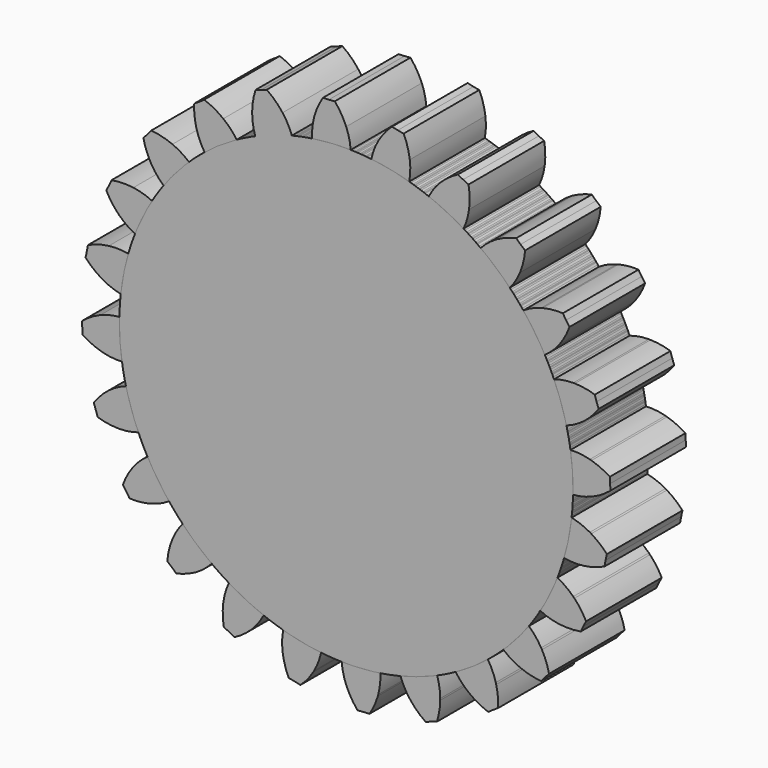
from build123d import *

# Parameters (mm, degrees)
F1_DEPTH = 25
F2_COUNT = 24
F2_ANGLE = 345


with BuildPart() as f1:
    # F0 (on Front) → F1 (new body)
    with BuildSketch(Plane.XZ):
        with BuildLine():
            ThreePointArc((-9.0111976673, 59.3194598475), (-39.1109200861, -45.5009442761), (60, 0))
            ThreePointArc((60, 0), (42.845546701, 42.0030847426), (1.1913624036, 59.9881709641))
            ThreePointArc((1.1913624036, 59.9881709641), (-1.3676565953, 59.9844106034), (-3.9241877538, 59.8715353943))
            ThreePointArc((-3.9241877538, 59.8715353943), (-6.4735806051, 59.6497506629), (-9.0111976673, 59.3194598475))
        make_face()
        with BuildLine():
            ThreePointArc((-8.4842024943, 64.4439159893), (-8.9485442404, 61.9023425791), (-9.0111976673, 59.3194598475))
            ThreePointArc((-9.0111976673, 59.3194598475), (-6.4735806051, 59.6497506629), (-3.9241877538, 59.8715353943))
            Line((-3.9241877538, 59.8715353943), (-4.2559103924, 64.9326448372))
            Line((-4.2559103924, 64.9326448372), (-8.3665646405, 64.8675885366))
            ThreePointArc((-8.3665646405, 64.8675885366), (-8.4266447953, 64.6561024583), (-8.4842024943, 64.4439159893))
        make_face()
        with BuildLine():
            Line((-8.3665646405, 64.8675885366), (-4.2559103924, 64.9326448372))
            Line((-4.2559103924, 64.9326448372), (-4.5749731638, 69.8006020322))
            ThreePointArc((-4.5749731638, 69.8006020322), (-5.361514281, 69.7570438044), (-6.1487762364, 69.7294238524))
            ThreePointArc((-6.1487762364, 69.7294238524), (-7.4344903349, 67.3791648533), (-8.3665646405, 64.8675885366))
        make_face()
        with BuildLine():
            Line((-4.2559103924, 64.9326448372), (0, 65))
            ThreePointArc((0, 65), (-1.3083979526, 67.5860266971), (-3.0053435778, 69.935455314))
            ThreePointArc((-3.0053435778, 69.935455314), (-3.7894755253, 69.8600806681), (-4.5749731638, 69.8006020322))
            Line((-4.5749731638, 69.8006020322), (-4.2559103924, 64.9326448372))
        make_face()
        with BuildLine():
            ThreePointArc((-3.9241877538, 59.8715353943), (-1.3676565953, 59.9844106034), (1.1913624036, 59.9881709641))
            ThreePointArc((1.1913624036, 59.9881709641), (0.7921111376, 62.5407788626), (0, 65))
            Line((0, 65), (-4.2559103924, 64.9326448372))
            Line((-4.2559103924, 64.9326448372), (-3.9241877538, 59.8715353943))
        make_face()
    extrude(amount=F1_DEPTH)


with BuildPart() as f2_1:
    # F2: instance of F1
    add(f1.part.rotate(Axis((0, -25, 0), (0, 1, 0)), 1 * F2_ANGLE / (F2_COUNT - 1)))


with BuildPart() as f2_2:
    # F2: instance of F1
    add(f1.part.rotate(Axis((0, -25, 0), (0, 1, 0)), 2 * F2_ANGLE / (F2_COUNT - 1)))


with BuildPart() as f2_3:
    # F2: instance of F1
    add(f1.part.rotate(Axis((0, -25, 0), (0, 1, 0)), 3 * F2_ANGLE / (F2_COUNT - 1)))


with BuildPart() as f2_4:
    # F2: instance of F1
    add(f1.part.rotate(Axis((0, -25, 0), (0, 1, 0)), 4 * F2_ANGLE / (F2_COUNT - 1)))


with BuildPart() as f2_5:
    # F2: instance of F1
    add(f1.part.rotate(Axis((0, -25, 0), (0, 1, 0)), 5 * F2_ANGLE / (F2_COUNT - 1)))


with BuildPart() as f2_6:
    # F2: instance of F1
    add(f1.part.rotate(Axis((0, -25, 0), (0, 1, 0)), 6 * F2_ANGLE / (F2_COUNT - 1)))


with BuildPart() as f2_7:
    # F2: instance of F1
    add(f1.part.rotate(Axis((0, -25, 0), (0, 1, 0)), 7 * F2_ANGLE / (F2_COUNT - 1)))


with BuildPart() as f2_8:
    # F2: instance of F1
    add(f1.part.rotate(Axis((0, -25, 0), (0, 1, 0)), 8 * F2_ANGLE / (F2_COUNT - 1)))


with BuildPart() as f2_9:
    # F2: instance of F1
    add(f1.part.rotate(Axis((0, -25, 0), (0, 1, 0)), 9 * F2_ANGLE / (F2_COUNT - 1)))


with BuildPart() as f2_10:
    # F2: instance of F1
    add(f1.part.rotate(Axis((0, -25, 0), (0, 1, 0)), 10 * F2_ANGLE / (F2_COUNT - 1)))


with BuildPart() as f2_11:
    # F2: instance of F1
    add(f1.part.rotate(Axis((0, -25, 0), (0, 1, 0)), 11 * F2_ANGLE / (F2_COUNT - 1)))


with BuildPart() as f2_12:
    # F2: instance of F1
    add(f1.part.rotate(Axis((0, -25, 0), (0, 1, 0)), 12 * F2_ANGLE / (F2_COUNT - 1)))


with BuildPart() as f2_13:
    # F2: instance of F1
    add(f1.part.rotate(Axis((0, -25, 0), (0, 1, 0)), 13 * F2_ANGLE / (F2_COUNT - 1)))


with BuildPart() as f2_14:
    # F2: instance of F1
    add(f1.part.rotate(Axis((0, -25, 0), (0, 1, 0)), 14 * F2_ANGLE / (F2_COUNT - 1)))


with BuildPart() as f2_15:
    # F2: instance of F1
    add(f1.part.rotate(Axis((0, -25, 0), (0, 1, 0)), 15 * F2_ANGLE / (F2_COUNT - 1)))


with BuildPart() as f2_16:
    # F2: instance of F1
    add(f1.part.rotate(Axis((0, -25, 0), (0, 1, 0)), 16 * F2_ANGLE / (F2_COUNT - 1)))


with BuildPart() as f2_17:
    # F2: instance of F1
    add(f1.part.rotate(Axis((0, -25, 0), (0, 1, 0)), 17 * F2_ANGLE / (F2_COUNT - 1)))


with BuildPart() as f2_18:
    # F2: instance of F1
    add(f1.part.rotate(Axis((0, -25, 0), (0, 1, 0)), 18 * F2_ANGLE / (F2_COUNT - 1)))


with BuildPart() as f2_19:
    # F2: instance of F1
    add(f1.part.rotate(Axis((0, -25, 0), (0, 1, 0)), 19 * F2_ANGLE / (F2_COUNT - 1)))


with BuildPart() as f2_20:
    # F2: instance of F1
    add(f1.part.rotate(Axis((0, -25, 0), (0, 1, 0)), 20 * F2_ANGLE / (F2_COUNT - 1)))


with BuildPart() as f2_21:
    # F2: instance of F1
    add(f1.part.rotate(Axis((0, -25, 0), (0, 1, 0)), 21 * F2_ANGLE / (F2_COUNT - 1)))


with BuildPart() as f2_22:
    # F2: instance of F1
    add(f1.part.rotate(Axis((0, -25, 0), (0, 1, 0)), 22 * F2_ANGLE / (F2_COUNT - 1)))


with BuildPart() as f2_23:
    # F2: instance of F1
    add(f1.part.rotate(Axis((0, -25, 0), (0, 1, 0)), 23 * F2_ANGLE / (F2_COUNT - 1)))


solid = Compound([f1.part, f2_1.part, f2_2.part, f2_3.part, f2_4.part, f2_5.part, f2_6.part, f2_7.part, f2_8.part, f2_9.part, f2_10.part, f2_11.part, f2_12.part, f2_13.part, f2_14.part, f2_15.part, f2_16.part, f2_17.part, f2_18.part, f2_19.part, f2_20.part, f2_21.part, f2_22.part, f2_23.part])
